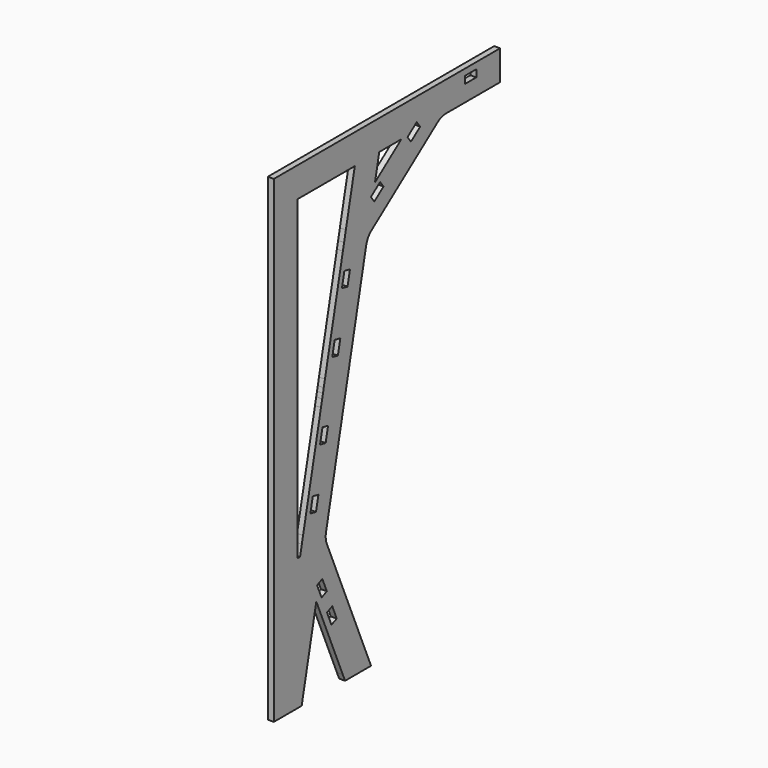
from build123d import *

# Parameters (mm, degrees)
F0_W     = 5.08
F0_H     = 2.54
F1_DEPTH = 2.1082
F2_R     = 0.762


with BuildPart() as f1:
    # F0 (on Right) → F1 (new body)
    with BuildSketch(Plane.YZ):
        with BuildLine():
            Line((0, 162.0091375), (0, 0))
            Line((0, 0), (12.335197777, 0))
            Line((12.335197777, 0), (18.8042013144, 29.896105485))
            Line((18.8042013144, 29.896105485), (30.5493542935, 2.3257501254))
            Line((30.5493542935, 2.3257501254), (31.5401391658, 0))
            Line((31.5401391658, 0), (31.5707651968, 0))
            Line((31.5707651968, 0), (40.8442968098, 0))
            Line((40.8442968098, 0), (20.5594925834, 47.616175108))
            Line((20.5594925834, 47.616175108), (39.5771112022, 135.5049402038))
            Line((39.5771112022, 135.5049402038), (73.5248959406, 160.7899383022))
            Line((73.5248959406, 160.7899383022), (100.203, 160.7899383022))
            Line((100.203, 160.7899383022), (100.203, 162.0091375))
            Line((100.203, 162.0091375), (82.1398573303, 162.0091375))
            ThreePointArc((82.1398573303, 162.0091375), (80.3438061061, 162.7530862758), (79.5998573303, 164.5491375))
            Line((79.5998573303, 164.5491375), (79.5998573303, 169.3418))
            Line((79.5998573303, 169.3418), (70.6874244764, 169.3418))
            Line((70.6874244764, 169.3418), (70.6874244764, 165.8480664454))
            Line((70.6874244764, 165.8480664454), (70.6874244764, 164.5491375))
            ThreePointArc((70.6874244764, 164.5491375), (70.0510915867, 162.8675752701), (68.4609272063, 162.0285589874))
            ThreePointArc((68.4609272063, 162.0285589874), (68.3044763435, 162.0139975214), (68.1474244764, 162.0091375))
            Line((68.1474244764, 162.0091375), (0, 162.0091375))
        make_face()
        Polygon((21.4843682503, 35.8535070154), (23.4753466245, 31.1799211209), (21.1385536773, 30.1844319338), (19.147575303, 34.8580178283), align=None, mode=Mode.SUBTRACT)
        Polygon((25.8665425285, 25.5668719827), (27.8575209028, 20.8932860882), (25.5207279555, 19.8977969011), (23.5297495813, 24.5713827956), align=None, mode=Mode.SUBTRACT)
        with BuildLine():
            Line((12.3986134924, 50.3752630702), (11.6175919588, 46.7658196656))
            Line((11.6175919588, 46.7658196656), (10.5918, 46.7658196656))
            Line((10.5918, 46.7658196656), (10.5918, 158.7579375))
            Line((10.5918, 158.7579375), (35.8507619547, 158.7579375))
            Line((35.8507619547, 158.7579375), (31.8897708968, 140.4524587956))
            Line((31.8897708968, 140.4524587956), (31.1087493632, 136.8430153909))
            Line((31.1087493632, 136.8430153909), (35.5475592049, 135.882533211))
            ThreePointArc((35.5475592049, 135.882533211), (37.1456481821, 134.7755682604), (37.4929253116, 132.8628062845))
            Line((37.4929253116, 132.8628062845), (29.5595533377, 96.1992113407))
            ThreePointArc((29.5595533377, 96.1992113407), (28.452588387, 94.6011223635), (26.5398264112, 94.2538452339))
            Line((26.5398264112, 94.2538452339), (22.1010165695, 95.2143274138))
            Line((22.1010165695, 95.2143274138), (21.7536814278, 93.6091392306))
            Line((21.7536814278, 93.6091392306), (21.4063462861, 92.0039510473))
            Line((21.4063462861, 92.0039510473), (25.8451561277, 91.0434688674))
            ThreePointArc((25.8451561277, 91.0434688674), (27.4432451049, 89.9365039168), (27.7905222345, 88.0237419409))
            Line((27.7905222345, 88.0237419409), (19.8571502605, 51.3601469971))
            ThreePointArc((19.8571502605, 51.3601469971), (18.7501853099, 49.7620580199), (16.837423334, 49.4147808903))
            Line((16.837423334, 49.4147808903), (12.3986134924, 50.3752630702))
        make_face(mode=Mode.SUBTRACT)
        Polygon((47.0613097153, 149.2568137468), (48.5785484084, 147.2197602993), (44.5044415132, 144.1852829132), (42.9872028202, 146.2223363607), align=None, mode=Mode.SUBTRACT)
        Polygon((44.8088104432, 150.074821282), (46.6876875952, 158.7579375), (56.4668125154, 158.7579375), align=None, mode=Mode.SUBTRACT)
        Polygon((63.2751536106, 161.3332132886), (64.7923923036, 159.296159841), (60.7182854085, 156.2616824549), (59.2010467154, 158.2987359025), align=None, mode=Mode.SUBTRACT)
        with BuildLine():
            Line((0, 164.5491375), (0, 162.0091375))
            Line((0, 162.0091375), (68.1474244764, 162.0091375))
            ThreePointArc((68.1474244764, 162.0091375), (68.3044763435, 162.0139975214), (68.4609272063, 162.0285589874))
            Line((68.4609272063, 162.0285589874), (69.6856973646, 162.9407926238))
            Line((69.6856973646, 162.9407926238), (68.1474244764, 165.0060867035))
            Line((68.1474244764, 165.0060867035), (68.1474244764, 164.5491375))
            Line((68.1474244764, 164.5491375), (55.1748093832, 164.5491375))
            Line((55.1748093832, 164.5491375), (50.0948093832, 164.5491375))
            Line((50.0948093832, 164.5491375), (10.3999171089, 164.5491375))
            Line((10.3999171089, 164.5491375), (5.3199171089, 164.5491375))
            Line((5.3199171089, 164.5491375), (0, 164.5491375))
        make_face()
        Polygon((0, 169.3418), (0, 164.5491375), (5.3199171089, 164.5491375), (5.3199171089, 167.0891375), (10.3999171089, 167.0891375), (10.3999171089, 164.5491375), (50.0948093832, 164.5491375), (50.0948093832, 167.0891375), (55.1748093832, 167.0891375), (55.1748093832, 164.5491375), (68.1474244764, 164.5491375), (68.1474244764, 165.0060867035), (68.1474244764, 169.3418), align=None)
        with Locations((7.8599171089, 165.8191375)):
            Rectangle(F0_W, F0_H)
        with BuildLine():
            Line((69.6856973646, 162.9407926238), (68.4609272063, 162.0285589874))
            ThreePointArc((68.4609272063, 162.0285589874), (70.0510915867, 162.8675752701), (70.6874244764, 164.5491375))
            Line((70.6874244764, 164.5491375), (70.6874244764, 165.8480664454))
            Line((70.6874244764, 165.8480664454), (70.6874244764, 169.3418))
            Line((70.6874244764, 169.3418), (68.1474244764, 169.3418))
            Line((68.1474244764, 169.3418), (68.1474244764, 165.0060867035))
            Line((68.1474244764, 165.0060867035), (69.6856973646, 162.9407926238))
        make_face()
        with Locations((52.6348093832, 165.8191375)):
            Rectangle(F0_W, F0_H)
        with BuildLine():
            Line((20.5594925834, 47.616175108), (40.8442968098, 0))
            Line((40.8442968098, 0), (43.053, 0))
            Line((43.053, 0), (23.4736756901, 45.9601445708))
            ThreePointArc((23.4736756901, 45.9601445708), (22.9941781878, 47.847708452), (23.1092917667, 49.7918185633))
            Line((23.1092917667, 49.7918185633), (40.8984089502, 132.0031391675))
            ThreePointArc((40.8984089502, 132.0031391675), (41.765080018, 134.0967787378), (43.3116785091, 135.7528217618))
            Line((43.3116785091, 135.7528217618), (72.5103326221, 157.500571119))
            ThreePointArc((72.5103326221, 157.500571119), (74.3053957564, 158.4354047741), (76.3034293547, 158.7579375))
            Line((76.3034293547, 158.7579375), (100.203, 158.7579375))
            Line((100.203, 158.7579375), (100.203, 160.7899383022))
            Line((100.203, 160.7899383022), (73.5248959406, 160.7899383022))
            Line((73.5248959406, 160.7899383022), (39.5771112022, 135.5049402038))
            Line((39.5771112022, 135.5049402038), (20.5594925834, 47.616175108))
        make_face()
        with BuildLine():
            Line((82.1398573303, 169.3418), (79.5998573303, 169.3418))
            Line((79.5998573303, 169.3418), (79.5998573303, 164.5491375))
            ThreePointArc((79.5998573303, 164.5491375), (80.3438061061, 162.7530862758), (82.1398573303, 162.0091375))
            Line((82.1398573303, 162.0091375), (100.203, 162.0091375))
            Line((100.203, 162.0091375), (100.203, 164.5491375))
            Line((100.203, 164.5491375), (89.6502663064, 164.5491375))
            Line((89.6502663064, 164.5491375), (84.5702663064, 164.5491375))
            Line((84.5702663064, 164.5491375), (82.1398573303, 164.5491375))
            Line((82.1398573303, 164.5491375), (82.1398573303, 169.3418))
        make_face()
        Polygon((100.203, 169.3418), (82.1398573303, 169.3418), (82.1398573303, 164.5491375), (84.5702663064, 164.5491375), (84.5702663064, 167.0891375), (89.6502663064, 167.0891375), (89.6502663064, 164.5491375), (100.203, 164.5491375), align=None)
        with BuildLine():
            Line((12.9357939022, 52.8578095868), (12.3986134924, 50.3752630702))
            Line((12.3986134924, 50.3752630702), (16.837423334, 49.4147808903))
            ThreePointArc((16.837423334, 49.4147808903), (18.7501853099, 49.7620580199), (19.8571502605, 51.3601469971))
            Line((19.8571502605, 51.3601469971), (27.7905222345, 88.0237419409))
            ThreePointArc((27.7905222345, 88.0237419409), (27.4432451049, 89.9365039168), (25.8451561277, 91.0434688674))
            Line((25.8451561277, 91.0434688674), (21.4063462861, 92.0039510473))
            Line((21.4063462861, 92.0039510473), (20.8691658762, 89.5214045307))
            Line((20.8691658762, 89.5214045307), (25.3079757178, 88.5609223508))
            Line((25.3079757178, 88.5609223508), (24.0175885553, 82.5974767434))
            Line((24.0175885553, 82.5974767434), (22.9432277355, 77.6323837102))
            Line((22.9432277355, 77.6323837102), (19.7419229759, 62.8377489213))
            Line((19.7419229759, 62.8377489213), (18.6675621562, 57.872655888))
            Line((18.6675621562, 57.872655888), (17.3746037439, 51.8973274069))
            Line((17.3746037439, 51.8973274069), (12.9357939022, 52.8578095868))
        make_face()
        Polygon((20.8691658762, 89.5214045307), (12.9357939022, 52.8578095868), (17.3746037439, 51.8973274069), (18.6675621562, 57.872655888), (16.1850156395, 58.4098362979), (17.2593764593, 63.3749293312), (19.7419229759, 62.8377489213), (22.9432277355, 77.6323837102), (20.4606812189, 78.16956412), (21.5350420386, 83.1346571533), (24.0175885553, 82.5974767434), (25.3079757178, 88.5609223508), align=None)
        with BuildLine():
            Line((35.5475592049, 135.882533211), (31.1087493632, 136.8430153909))
            Line((31.1087493632, 136.8430153909), (30.5715689534, 134.3604688743))
            Line((30.5715689534, 134.3604688743), (35.010378795, 133.3999866944))
            Line((35.010378795, 133.3999866944), (33.7174203827, 127.4246582133))
            Line((33.7174203827, 127.4246582133), (32.643059563, 122.45956518))
            Line((32.643059563, 122.45956518), (29.4417548033, 107.6649303911))
            Line((29.4417548033, 107.6649303911), (28.3673939836, 102.6998373579))
            Line((28.3673939836, 102.6998373579), (27.077006821, 96.7363917505))
            Line((27.077006821, 96.7363917505), (22.6381969794, 97.6968739305))
            Line((22.6381969794, 97.6968739305), (22.1010165695, 95.2143274138))
            Line((22.1010165695, 95.2143274138), (26.5398264112, 94.2538452339))
            ThreePointArc((26.5398264112, 94.2538452339), (28.452588387, 94.6011223635), (29.5595533377, 96.1992113407))
            Line((29.5595533377, 96.1992113407), (37.4929253116, 132.8628062845))
            ThreePointArc((37.4929253116, 132.8628062845), (37.1456481821, 134.7755682604), (35.5475592049, 135.882533211))
        make_face()
        Polygon((35.010378795, 133.3999866944), (30.5715689534, 134.3604688743), (22.6381969794, 97.6968739305), (27.077006821, 96.7363917505), (28.3673939836, 102.6998373579), (25.884847467, 103.2370177677), (26.9592082867, 108.202110801), (29.4417548033, 107.6649303911), (32.643059563, 122.45956518), (30.1605130463, 122.9967455899), (31.2348738661, 127.9618386231), (33.7174203827, 127.4246582133), align=None)
    extrude(amount=F1_DEPTH)

    # F2
    f2_edges = [f1.edges().sort_by_distance(p)[0] for p in [
        (0, 57.911006, 146.626696),
        (0, 33.263338, 22.980072),
        (0, 22.994178, 47.847708),
        (0, 32.00385, 90.897479),
        (0, 41.76508, 134.096779),
        (0, 74.305396, 158.435405),
        (0, 88.253215, 158.757937),
    ]]
    fillet(f2_edges, radius=F2_R)


solid = f1.part
